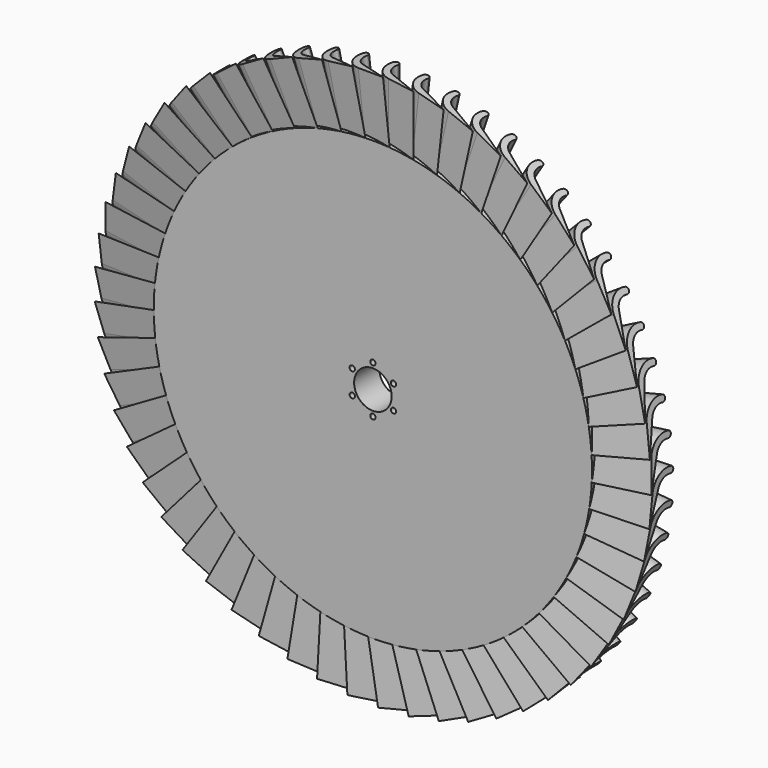
from build123d import *

# Parameters (mm, degrees)
F0_R            = 175
F1_DEPTH        = 12.5
F4_DEPTH        = 220
F4_COPIES_COUNT = 57
F3_R            = 15
F5_DEPTH        = 25.0010001007
F7_D            = 4.2
F7_COPIES_COUNT = 6


# Not quite as in the source:
# - a pattern or mirror of a feature is missing from the dataset's text; its kind, count and spacing are read off the source's solid


with BuildPart() as f1:
    # F0 (on Front) → F1 (new body, symmetric)
    with BuildSketch(Plane.XZ):
        Circle(F0_R)
    extrude(amount=F1_DEPTH, both=True)

    # F2 (on Top) → F4 (join)
    with BuildSketch(Plane.XY):
        with BuildLine():
            ThreePointArc((2.4038647175, 9.3133891788), (2.4758495303, 9.6533458451), (2.5, 10))
            ThreePointArc((2.5, 10), (0.3809030219, 12.470812192), (-2.3839303103, 10.7529118644))
            ThreePointArc((-2.3839303103, 10.7529118644), (-0.719830352, 7.605872964), (2.4038647175, 9.3133891788))
        make_face()
        with BuildLine():
            ThreePointArc((2.4038647175, 9.3133891788), (-0.719830352, 7.605872964), (-2.3839303103, 10.7529118644))
            ThreePointArc((-2.3839303103, 10.7529118644), (-0.8850167679, -1.577399345), (9.3941042981, -8.5504178046))
            Line((9.3941042981, -8.5504178046), (32.5169990791, -12.5))
            Line((32.5169990791, -12.5), (8.2732576535, -2.7048926517))
            ThreePointArc((8.2732576535, -2.7048926517), (3.0336482756, 2.1785932205), (2.4038647175, 9.3133891788))
        make_face()
    f4 = extrude(amount=F4_DEPTH)

    # F4_copies: F4 ×57 about axis
    f4_copies_axis = Axis((0, 0, 0), (0, 1, 0))
    for i in range(1, F4_COPIES_COUNT):
        add(f4.rotate(f4_copies_axis, i * 360 / F4_COPIES_COUNT))

    # F3 (on face) → F5 (cut, through all)
    with BuildSketch(Plane.XZ.offset(12.5)):
        Circle(F3_R)
    extrude(amount=-F5_DEPTH, mode=Mode.SUBTRACT)

    # F7 (through all)
    with Locations(Plane.XZ.offset(12.5)):
        with Locations((0, 19)):
            f7 = Hole(F7_D / 2)

    # F7_copies: F7 ×6 about axis
    f7_copies_axis = Axis((0, 0, 0), (0, 1, 0))
    for i in range(1, F7_COPIES_COUNT):
        add(f7.rotate(f7_copies_axis, i * 360 / F7_COPIES_COUNT), mode=Mode.SUBTRACT)


solid = f1.part
